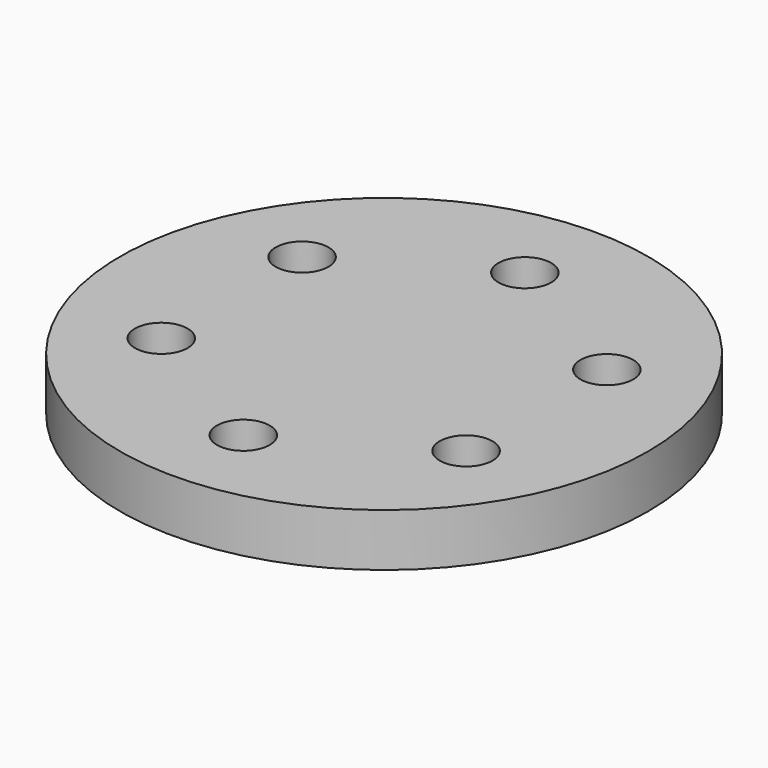
from build123d import *

# Parameters (mm, degrees)
F2_R            = 60
F3_DEPTH        = 12
F4_R            = 6
F5_DEPTH        = 12.001
F5_COPIES_COUNT = 6


# Not quite as in the source:
# - a pattern or mirror of a feature is missing from the dataset's text; its kind, count and spacing are read off the source's solid


with BuildPart() as f3:
    # F2 (on Top) → F3 (new body)
    with BuildSketch(Plane.XY):
        Circle(F2_R)
    extrude(amount=F3_DEPTH)

    # F4 (on face) → F5 (cut, through all)
    with BuildSketch(Plane.XY.offset(12)):
        with Locations((0, 40)):
            Circle(F4_R)
    f5 = extrude(amount=-F5_DEPTH, mode=Mode.SUBTRACT)

    # F5_copies: F5 ×6 about axis
    f5_copies_axis = Axis((0, 0, 0), (0, 0, 1))
    for i in range(1, F5_COPIES_COUNT):
        add(f5.rotate(f5_copies_axis, i * 360 / F5_COPIES_COUNT), mode=Mode.SUBTRACT)


solid = f3.part
